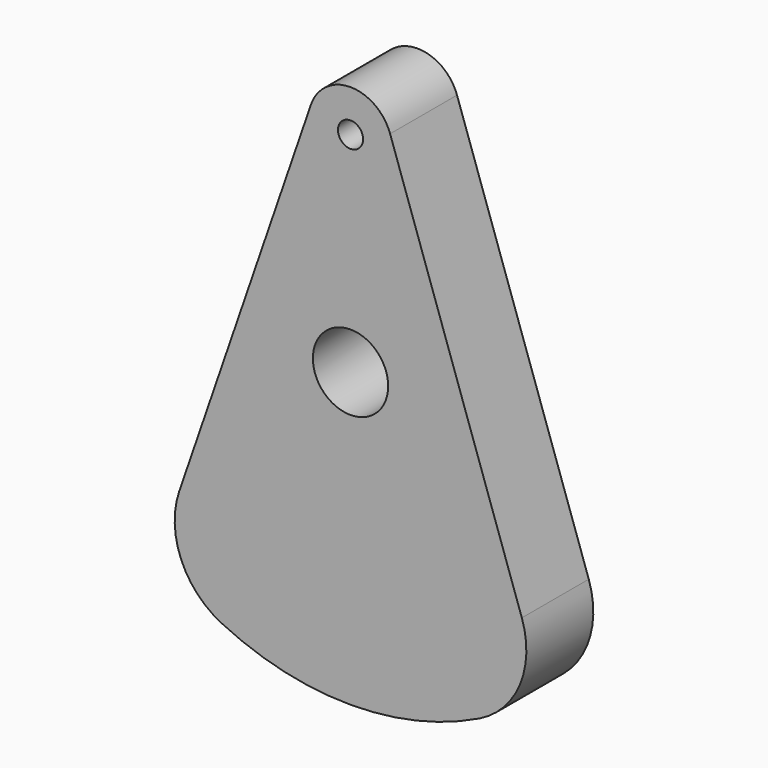
from build123d import *

# Parameters (mm, degrees)
F1_DEPTH = 1
F2_R     = 0.9
F2_R_2   = 0.3
F3_DEPTH = 2.001
F4_R     = 2


# Not quite as in the source:
# - a feature names something its author has since deleted; it is built from what else it names


with BuildPart() as f1:
    # F0 (on Front) → F1 (new body, symmetric)
    with BuildSketch(Plane.XZ):
        with BuildLine():
            ThreePointArc((-0.9457076356, 5.3250185657), (-0.1647609851, 4.0136664774), (1, 5))
            ThreePointArc((1, 5), (0.9863335226, 5.1647609851), (0.9457076356, 5.3250185657))
            ThreePointArc((0.9457076356, 5.3250185657), (0, 6), (-0.9457076356, 5.3250185657))
        make_face()
        with BuildLine():
            ThreePointArc((0.9457076356, 5.3250185657), (0.9863335226, 5.1647609851), (1, 5))
            ThreePointArc((1, 5), (-0.1647609851, 4.0136664774), (-0.9457076356, 5.3250185657))
            Line((-0.9457076356, 5.3250185657), (-4.5916600475, -5.2836216754))
            ThreePointArc((-4.5916600475, -5.2836216754), (0, -6.9972097643), (4.5916600475, -5.2836216754))
            Line((4.5916600475, -5.2836216754), (0.9457076356, 5.3250185657))
        make_face()
    extrude(amount=F1_DEPTH, both=True)

    # F2 (on face) → F3 (cut, through all)
    with BuildSketch(Plane.XZ.offset(1)):
        Circle(F2_R)
        with Locations((0, 5)):
            Circle(F2_R_2)
    extrude(amount=-F3_DEPTH, mode=Mode.SUBTRACT)

    # F4
    f4_edges = [f1.edges().sort_by_distance(p)[0] for p in [
        (4.59166, 0, -5.283622),
        (-4.59166, 0, -5.283622),
    ]]
    fillet(f4_edges, radius=F4_R)


solid = f1.part
